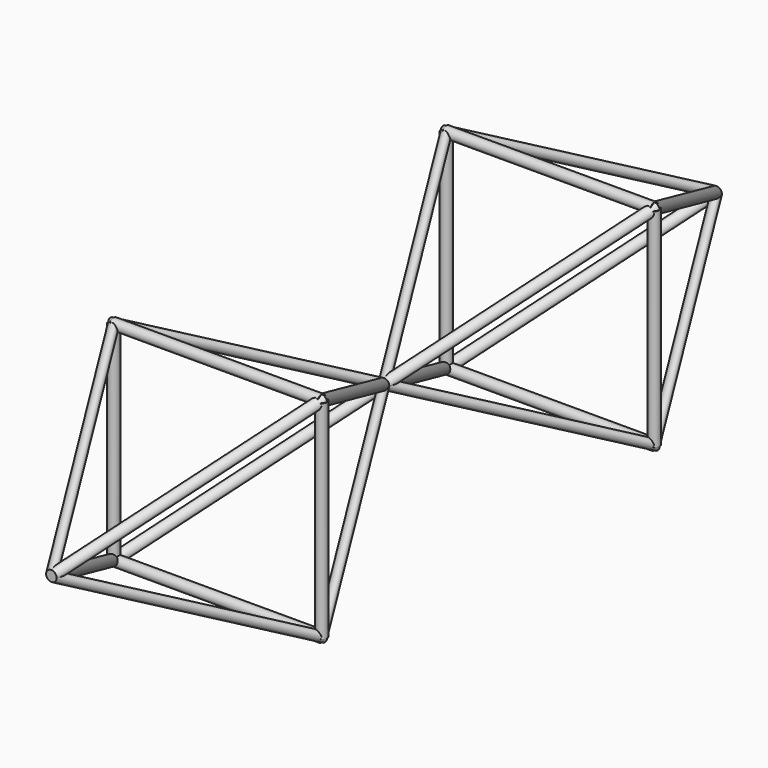
from build123d import *

# Parameters (mm, degrees)
F4_R      = 12.7
F6_COUNT  = 4
F6_ANGLE  = 270
F8_R      = 12.7
F9_DEPTH  = 250
F10_COUNT = 4
F10_ANGLE = 270


with BuildPart() as f5:
    # F5: sweep along a path in F3
    with BuildLine(Plane(origin=(0, 0, 0), x_dir=(0.7071067812, 0, 0.7071067812), z_dir=(0.7071067812, 0, -0.7071067812))) as f5_path:
        Line((0, 500), (353.5533905933, 0))
    # F4 (on face) → F5 (sweep)
    with BuildSketch(Plane.XZ):
        with Locations((250, 250)):
            Circle(F4_R)
    sweep(path=f5_path.line)


with BuildPart() as f6_1:
    # F6: instance of F5
    add(f5.part.rotate(Axis((0, -250, 0), (0, -1, 0)), 1 * F6_ANGLE / (F6_COUNT - 1)))


with BuildPart() as f6_2:
    # F6: instance of F5
    add(f5.part.rotate(Axis((0, -250, 0), (0, -1, 0)), 2 * F6_ANGLE / (F6_COUNT - 1)))


with BuildPart() as f6_3:
    # F6: instance of F5
    add(f5.part.rotate(Axis((0, -250, 0), (0, -1, 0)), 3 * F6_ANGLE / (F6_COUNT - 1)))


with BuildPart() as f7_1:
    # F7: instance of F6_1
    add(f6_1.part.mirror(Plane.XZ))


with BuildPart() as f7_2:
    # F7: instance of F6_3
    add(f6_3.part.mirror(Plane.XZ))


with BuildPart() as f7_3:
    # F7: instance of F5
    add(f5.part.mirror(Plane.XZ))


with BuildPart() as f7_4:
    # F7: instance of F6_2
    add(f6_2.part.mirror(Plane.XZ))


with BuildPart() as f9:
    # F8 (on Right) → F9 (new body, symmetric)
    with BuildSketch(Plane.YZ):
        with Locations((0, 250)):
            Circle(F8_R)
    extrude(amount=F9_DEPTH, both=True)


with BuildPart() as f10_1:
    # F10: instance of F9
    add(f9.part.rotate(Axis((0, -250, 0), (0, -1, 0)), 1 * F10_ANGLE / (F10_COUNT - 1)))


with BuildPart() as f10_2:
    # F10: instance of F9
    add(f9.part.rotate(Axis((0, -250, 0), (0, -1, 0)), 2 * F10_ANGLE / (F10_COUNT - 1)))


with BuildPart() as f10_3:
    # F10: instance of F9
    add(f9.part.rotate(Axis((0, -250, 0), (0, -1, 0)), 3 * F10_ANGLE / (F10_COUNT - 1)))


with BuildPart() as f12_1:
    # F12: instance of F7_1
    add(f7_1.part.mirror(Plane.XZ.offset(500)))


with BuildPart() as f12_2:
    # F12: instance of F6_1
    add(f6_1.part.mirror(Plane.XZ.offset(500)))


with BuildPart() as f12_3:
    # F12: instance of F6_3
    add(f6_3.part.mirror(Plane.XZ.offset(500)))


with BuildPart() as f12_4:
    # F12: instance of F10_3
    add(f10_3.part.mirror(Plane.XZ.offset(500)))


with BuildPart() as f12_5:
    # F12: instance of F5
    add(f5.part.mirror(Plane.XZ.offset(500)))


with BuildPart() as f12_6:
    # F12: instance of F7_3
    add(f7_3.part.mirror(Plane.XZ.offset(500)))


with BuildPart() as f12_7:
    # F12: instance of F6_2
    add(f6_2.part.mirror(Plane.XZ.offset(500)))


with BuildPart() as f12_8:
    # F12: instance of F7_4
    add(f7_4.part.mirror(Plane.XZ.offset(500)))


with BuildPart() as f12_9:
    # F12: instance of F7_2
    add(f7_2.part.mirror(Plane.XZ.offset(500)))


with BuildPart() as f12_10:
    # F12: instance of F9
    add(f9.part.mirror(Plane.XZ.offset(500)))


with BuildPart() as f12_11:
    # F12: instance of F10_1
    add(f10_1.part.mirror(Plane.XZ.offset(500)))


with BuildPart() as f12_12:
    # F12: instance of F10_2
    add(f10_2.part.mirror(Plane.XZ.offset(500)))


solid = Compound([f5.part, f6_1.part, f6_2.part, f6_3.part, f7_1.part, f7_2.part, f7_3.part, f7_4.part, f9.part, f10_1.part, f10_2.part, f10_3.part, f12_1.part, f12_2.part, f12_3.part, f12_4.part, f12_5.part, f12_6.part, f12_7.part, f12_8.part, f12_9.part, f12_10.part, f12_11.part, f12_12.part])
